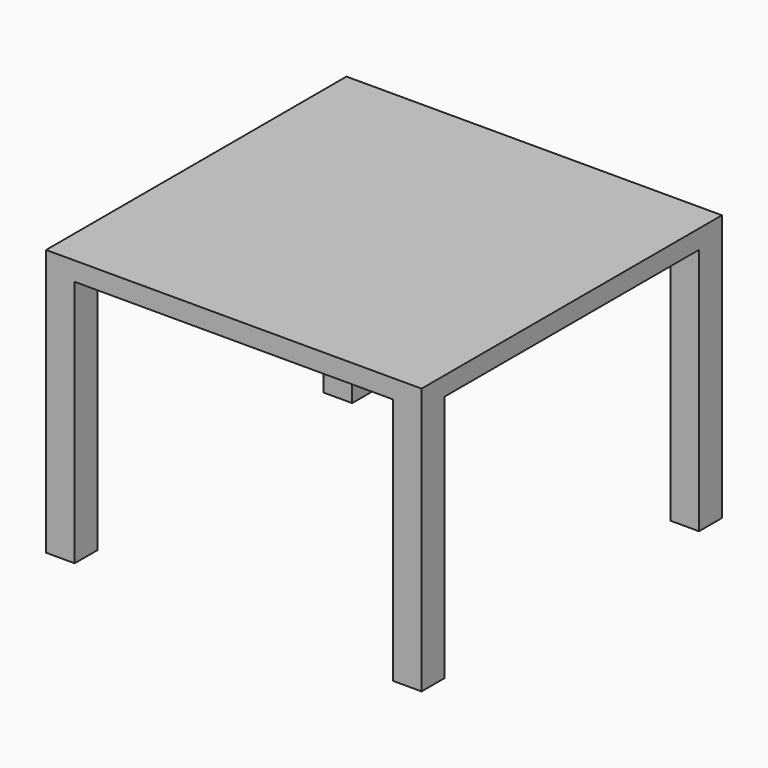
from build123d import *

# Parameters (mm, degrees)
F0_W         = 1000
F0_H         = 1000
F1_DEPTH     = 25
F2_W         = 76.2
F2_H         = 76.2
F3_DEPTH     = 660
F4_TEXT_SIZE = 163.394980877
F5_DEPTH     = 19.05


# Not quite as in the source:
# - Text() gives the source's letters only with a copy of the font that has no kerning and outlines rounded to 1/6400 em; it was checked with that copy


with BuildPart() as f1:
    # F0 (on Top) → F1 (new body, symmetric)
    with BuildSketch(Plane.XY):
        Rectangle(F0_W, F0_H)
    extrude(amount=F1_DEPTH, both=True)

    # F2 (on face) → F3 (join)
    with BuildSketch(Plane(origin=(0, 0, -25), x_dir=(1, 0, 0), z_dir=(0, 0, -1))):
        with Locations((-461.9, 461.9)):
            Rectangle(F2_W, F2_H)
        with Locations((-461.9, -461.9)):
            Rectangle(F2_W, F2_H)
        with Locations((461.9, -461.9)):
            Rectangle(F2_W, F2_H)
        with Locations((461.9, 461.9)):
            Rectangle(F2_W, F2_H)
    extrude(amount=F3_DEPTH)

    # F4 (on Top) → F5 (cut, symmetric)
    with BuildSketch(Plane.XY):
        with Locations((-487.3, 45.0581638815)):
            Text('Colin Smeels', F4_TEXT_SIZE, font='Open Sans', text_align=(TextAlign.LEFT, TextAlign.BOTTOM))
    extrude(amount=F5_DEPTH, both=True, mode=Mode.SUBTRACT)


solid = f1.part
